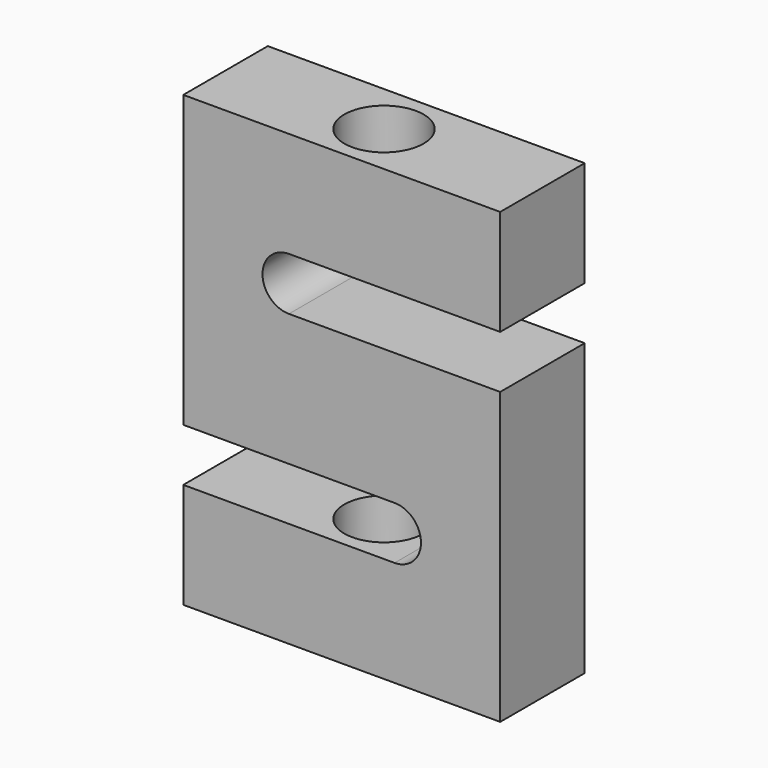
from build123d import *

# Parameters (mm, degrees)
F1_DEPTH = 25.4
F2_R     = 9.525
F3_DEPTH = 25.4


# Not quite as in the source:
# - a pattern or mirror of a feature is missing from the dataset's text; its kind, count and spacing are read off the source's solid


with BuildPart() as f1:
    # F0 (on Front) → F1 (new body)
    with BuildSketch(Plane.XZ):
        with BuildLine():
            Line((38.1, 53.975), (-38.1, 53.975))
            Line((-38.1, 53.975), (-38.1, -15.875))
            Line((-38.1, -15.875), (12.7, -15.875))
            ThreePointArc((12.7, -15.875), (19.05, -22.225), (12.7, -28.575))
            Line((12.7, -28.575), (-38.1, -28.575))
            Line((-38.1, -28.575), (-38.1, -53.975))
            Line((-38.1, -53.975), (38.1, -53.975))
            Line((38.1, -53.975), (38.1, 15.875))
            Line((38.1, 15.875), (-12.7, 15.875))
            ThreePointArc((-12.7, 15.875), (-19.05, 22.225), (-12.7, 28.575))
            Line((-12.7, 28.575), (38.1, 28.575))
            Line((38.1, 28.575), (38.1, 53.975))
        make_face()
    extrude(amount=F1_DEPTH)

    # F2 (on face) → F3 (cut, through all)
    with BuildSketch(Plane.XY.offset(53.975)):
        with Locations((0, -12.7)):
            Circle(F2_R)
    f3 = extrude(amount=-F3_DEPTH, mode=Mode.SUBTRACT)

    # F3_copies: F3 across plane
    add(f3.mirror(Plane(origin=(0, 0, 0), x_dir=(-1, 0, 0), z_dir=(0, 0, -1))), mode=Mode.SUBTRACT)


solid = f1.part
